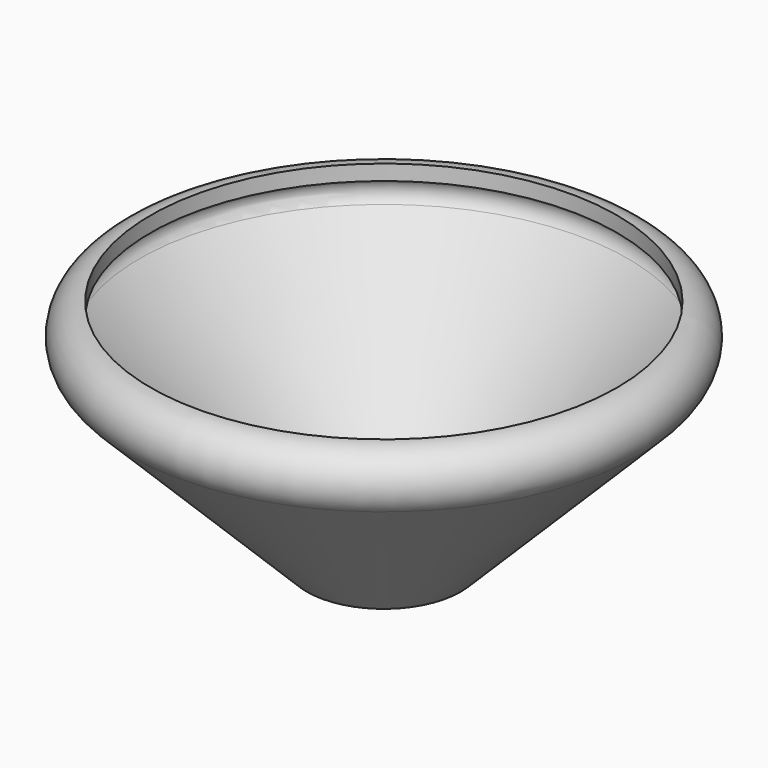
from build123d import *

# Parameters (mm, degrees)
F2_R = 5.08
F3_T = -2.54
F5_D = 25.4


# Not quite as in the source:
# - a shell that OpenCascade refuses in one call is made with other operations: the cavity is built on its own and cut out


with BuildPart() as f1:
    # F0 (on Front) → F1 (revolve)
    with BuildSketch(Plane.XZ):
        Polygon((0, 50.8), (0, 0), (50.8, 50.8), align=None)
    revolve(axis=Axis((0, 0, 25.4), (0, 0, 1)))

    # F2
    f2_edges = [f1.edges().sort_by_distance(p)[0] for p in [
        (-50.8, 0, 50.8),
    ]]
    fillet(f2_edges, radius=F2_R)

    # F3: a shell. OpenCascade refuses it in one call, so the cavity is built on its own and cut out:
    # the body offset inwards by the wall thickness, plus a prism from it out through each open face.
    f3_core = offset(f1.part, amount=F3_T, mode=Mode.PRIVATE)
    f3_exits = [f3_core.faces().sort_by_distance(p)[0] for p in [
        (0, 0, 48.26),
    ]]
    add(f3_core, mode=Mode.SUBTRACT)
    extrude(f3_exits, amount=-F3_T, mode=Mode.SUBTRACT)

    # F5 (through all)
    with Locations(Plane(origin=(0, 0, 0), x_dir=(1, 0, 0), z_dir=(0, 0, -1))):
        with Locations((0, 0)):
            Hole(F5_D / 2)


solid = f1.part
